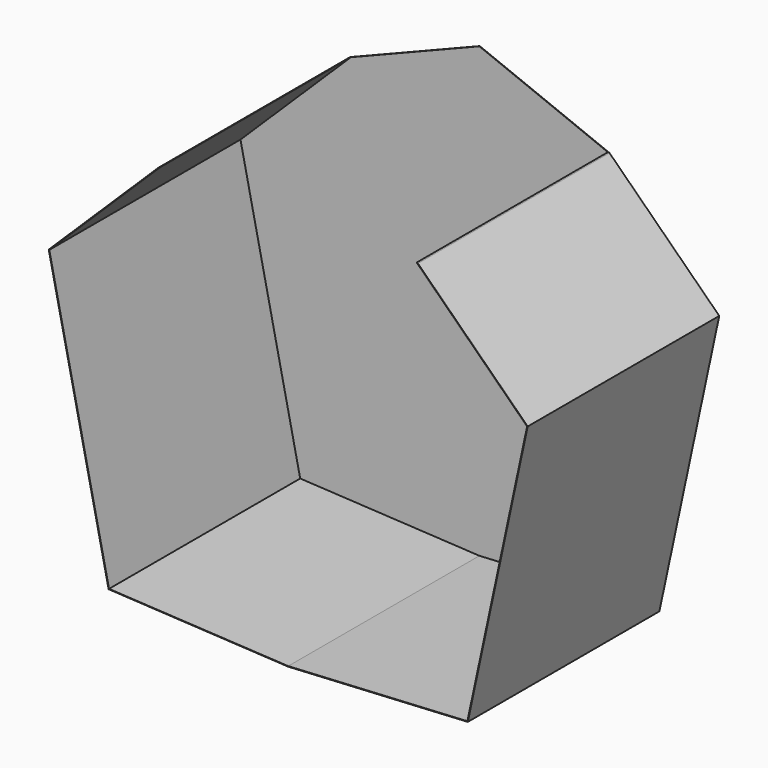
from build123d import *

# Parameters (mm, degrees)
F1_DEPTH = 1200
F2_T     = -2.5


# Not quite as in the source:
# - the program builds the solid bodies; features that only make, move or delete a surface that nothing else refers to are left out


with BuildPart() as f1:
    # F0 (on Front) → F1 (new body)
    with BuildSketch(Plane.XZ):
        with BuildLine():
            Line((1200, 700), (64.7834175674, 37.7903269143))
            ThreePointArc((64.7834175674, 37.7903269143), (72.4008160091, 19.5734984411), (75, 0))
            ThreePointArc((75, 0), (70.9319827149, -24.3650123769), (59.1692312499, -46.0868969805))
            Line((59.1692312499, -46.0868969805), (900, -701.0097377681))
            Line((900, -701.0097377681), (1200, 700))
        make_face()
        with BuildLine():
            Line((0, -750), (900, -701.0097377681))
            Line((900, -701.0097377681), (59.1692312499, -46.0868969805))
            ThreePointArc((59.1692312499, -46.0868969805), (32.9278205053, -67.3851514562), (0, -75))
            Line((0, -75), (0, -750))
        make_face()
        with BuildLine():
            ThreePointArc((0, -75), (-32.9278205053, -67.3851514562), (-59.1692312499, -46.0868969805))
            Line((-59.1692312499, -46.0868969805), (-900, -701.0097377681))
            Line((-900, -701.0097377681), (0, -750))
            Line((0, -750), (0, -75))
        make_face()
        with BuildLine():
            ThreePointArc((-59.1692312499, -46.0868969805), (-74.8325594864, -5.0087963342), (-64.7834175674, 37.7903269143))
            Line((-64.7834175674, 37.7903269143), (-1200, 700))
            Line((-1200, 700), (-900, -701.0097377681))
            Line((-900, -701.0097377681), (-59.1692312499, -46.0868969805))
        make_face()
        with BuildLine():
            ThreePointArc((-64.7834175674, 37.7903269143), (-51.8193989205, 54.2194604872), (-34.8205403037, 66.426876887))
            Line((-34.8205403037, 66.426876887), (-650, 1240))
            Line((-650, 1240), (-1200, 700))
            Line((-1200, 700), (-64.7834175674, 37.7903269143))
        make_face()
        with BuildLine():
            ThreePointArc((-34.8205403037, 66.426876887), (-17.9302012464, 72.8251871488), (0, 75))
            Line((0, 75), (0, 1500))
            Line((0, 1500), (-650, 1240))
            Line((-650, 1240), (-34.8205403037, 66.426876887))
        make_face()
        with BuildLine():
            Line((0, 1500), (0, 75))
            ThreePointArc((0, 75), (17.9302012464, 72.8251871488), (34.8205403037, 66.426876887))
            Line((34.8205403037, 66.426876887), (650, 1240))
            Line((650, 1240), (0, 1500))
        make_face()
        with BuildLine():
            Line((650, 1240), (34.8205403037, 66.426876887))
            ThreePointArc((34.8205403037, 66.426876887), (51.8193989205, 54.2194604872), (64.7834175674, 37.7903269143))
            Line((64.7834175674, 37.7903269143), (1200, 700))
            Line((1200, 700), (650, 1240))
        make_face()
        with BuildLine():
            ThreePointArc((34.8205403037, 66.426876887), (17.9302012464, 72.8251871488), (0, 75))
            ThreePointArc((0, 75), (-17.9302012464, 72.8251871488), (-34.8205403037, 66.426876887))
            ThreePointArc((-34.8205403037, 66.426876887), (-51.8193989205, 54.2194604872), (-64.7834175674, 37.7903269143))
            ThreePointArc((-64.7834175674, 37.7903269143), (-74.8325594864, -5.0087963342), (-59.1692312499, -46.0868969805))
            ThreePointArc((-59.1692312499, -46.0868969805), (-32.9278205053, -67.3851514562), (0, -75))
            ThreePointArc((0, -75), (32.9278205053, -67.3851514562), (59.1692312499, -46.0868969805))
            ThreePointArc((59.1692312499, -46.0868969805), (70.9319827149, -24.3650123769), (75, 0))
            ThreePointArc((75, 0), (72.4008160091, 19.5734984411), (64.7834175674, 37.7903269143))
            ThreePointArc((64.7834175674, 37.7903269143), (51.8193989205, 54.2194604872), (34.8205403037, 66.426876887))
        make_face()
    extrude(amount=F1_DEPTH)

    # F2
    f2_openings = [f1.faces().sort_by_distance(p)[0] for p in [
        (-325, -600, 1370),
        (325, -600, 1370),
        (0, -1200, 296.454391),
    ]]
    offset(amount=F2_T, openings=f2_openings)


solid = f1.part
